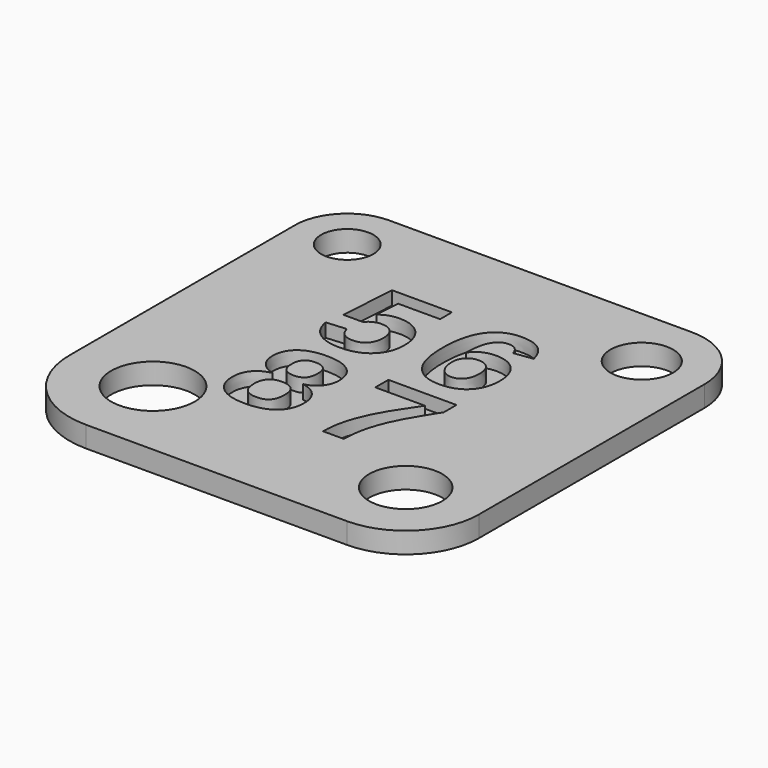
from build123d import *

# Parameters (mm, degrees)
F1_DEPTH     = 2
F2_TEXT_SIZE = 13.8888888889
F3_DEPTH     = 1.3
F2_R         = 2.5
F2_R_2       = 3
F2_R_3       = 3.5
F2_R_4       = 4
F4_DEPTH     = 25


# Not quite as in the source:
# - Text() gives the source's letters only with a copy of the font that has no kerning and outlines rounded to 1/6400 em; it was checked with that copy


with BuildPart() as f1:
    # F0 (on Top) → F1 (new body)
    with BuildSketch(Plane.XY):
        with BuildLine():
            Line((14, 20), (-15, 20))
            ThreePointArc((-15, 20), (-18.5355339059, 18.5355339059), (-20, 15))
            Line((-20, 15), (-20, -12))
            ThreePointArc((-20, -12), (-17.6568542495, -17.6568542495), (-12, -20))
            Line((-12, -20), (13, -20))
            ThreePointArc((13, -20), (17.9497474683, -17.9497474683), (20, -13))
            Line((20, -13), (20, 14))
            ThreePointArc((20, 14), (18.2426406871, 18.2426406871), (14, 20))
        make_face()
    extrude(amount=F1_DEPTH)

    # F2 (on face) → F3 (cut)
    with BuildSketch(Plane.XY.offset(2)):
        with Locations((-8.80078125, 1.75)):
            Text('5', F2_TEXT_SIZE, font='Arimo', font_style=FontStyle.BOLD, text_align=(TextAlign.LEFT, TextAlign.BOTTOM))
        with Locations((0.5, 1.75)):
            Text('6', F2_TEXT_SIZE, font='Arimo', font_style=FontStyle.BOLD, text_align=(TextAlign.LEFT, TextAlign.BOTTOM))
        with Locations((0.5, -9.75)):
            Text('7', F2_TEXT_SIZE, font='Arimo', font_style=FontStyle.BOLD, text_align=(TextAlign.LEFT, TextAlign.BOTTOM))
        with Locations((-8.76171875, -9.75)):
            Text('8', F2_TEXT_SIZE, font='Arimo', font_style=FontStyle.BOLD, text_align=(TextAlign.LEFT, TextAlign.BOTTOM))
    extrude(amount=-F3_DEPTH, mode=Mode.SUBTRACT)

    # F2 (on face) → F4 (cut)
    with BuildSketch(Plane.XY.offset(2)):
        with Locations((-15, 15)):
            Circle(F2_R)
        with Locations((14, 14)):
            Circle(F2_R_2)
        with Locations((13, -13)):
            Circle(F2_R_3)
        with Locations((-12, -12)):
            Circle(F2_R_4)
    extrude(amount=-F4_DEPTH, mode=Mode.SUBTRACT)


solid = f1.part
